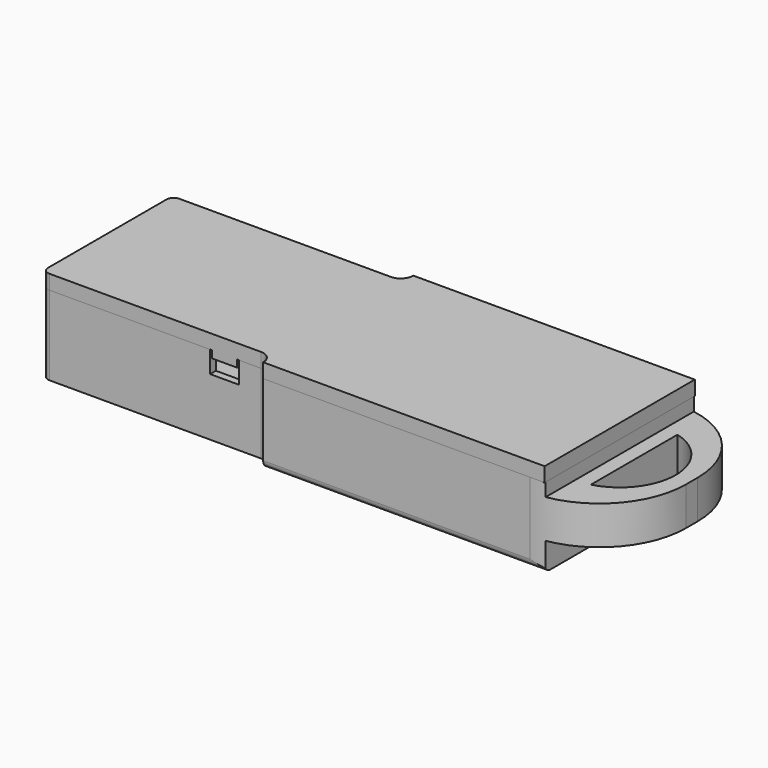
from build123d import *

# Parameters (mm, degrees)
F0_W         = 31
F0_H         = 17.5
F0_W_2       = 1
F1_DEPTH     = 8.5
F2_T         = 2.5
F3_W         = 1
F3_H         = 1
F4_DEPTH     = 6.5
F5_R         = 1
F6_W         = 9.5
F6_H         = 6
F8_DEPTH     = 1.5
F7_W         = 4
F7_H         = 4
F9_DEPTH     = 2
F11_DEPTH    = 2
F13_DEPTH    = 2
F14_R        = 1
F15_R        = 1.7
F15_2_R      = 1.7
F17_DEPTH    = 1.75
F18_W        = 12.5
F18_H        = 7.25
F19_DEPTH    = 3
F20_W        = 1.25
F20_H        = 12
F21_DEPTH    = 2.25
F22_W        = 3.5
F22_H        = 1
F23_DEPTH    = 1
F24_W        = 1
F24_H        = 4
F25_DEPTH    = 2
F26_W        = 2
F26_H        = 4
F27_DEPTH    = 1
F28_SIZE     = 0.99999
F29_W        = 6
F29_H        = 2
F30_DEPTH    = 0.25
F32_DEPTH    = 10
F33_T1_DEPTH = 65.3331902927
F35_DEPTH    = 10


# Not quite as in the source:
# - a fillet or chamfer that OpenCascade refuses, or shapes differently, is made with other operations: its cross-section is extruded or revolved along the edge and cut away or added
# - a fillet or chamfer is up to 0.001 mm smaller than in the source, because OpenCascade refuses the exact size


with BuildPart() as f1:
    # F0 (on Top) → F1 (new body)
    with BuildSketch(Plane.XY):
        Rectangle(F0_W, F0_H)
        with Locations((16, 0)):
            Rectangle(F0_W_2, F0_H)
        Polygon((16.5, 10.5), (16.5, 8.75), (16.5, -8.75), (16.5, -10.5), (50.5, -10.5), (50.5, 10.5), align=None)
    extrude(amount=F1_DEPTH)

    # F2
    f2_openings = [f1.faces().sort_by_distance(p)[0] for p in [
        (18.994505, 0, 8.5),
    ]]
    offset(amount=F2_T, openings=f2_openings, kind=Kind.INTERSECTION)

    # F3 (on face) → F4 (join)
    with BuildSketch(Plane.XY):
        with Locations((16, 4.5)):
            Rectangle(F3_W, F3_H)
        with Locations((16, 1.5)):
            Rectangle(F3_W, F3_H)
        with Locations((16, -1.5)):
            Rectangle(F3_W, F3_H)
        with Locations((16, -4.5)):
            Rectangle(F3_W, F3_H)
    extrude(amount=F4_DEPTH)

    # F5
    f5_edges = [f1.edges().sort_by_distance(p)[0] for p in [
        (-18, 11.25, 3),
        (-18, -11.25, 3),
        (33.5, -13, -2.5),
        (33.5, 13, -2.5),
    ]]
    fillet(f5_edges, radius=F5_R)

    # F6 (on face) → F8 (cut, symmetric)
    with BuildSketch(Plane(origin=(0, -8.75, 0), x_dir=(-1, 0, 0), z_dir=(0, 1, 0))):
        with Locations((-7.25, 7.5)):
            Rectangle(F6_W, F6_H)
    extrude(amount=F8_DEPTH, both=True, mode=Mode.SUBTRACT)

    # F7 (on face) → F9 (cut, symmetric)
    with BuildSketch(Plane.XZ.offset(11.25)):
        with Locations((7.25, 7.5)):
            Rectangle(F7_W, F7_H)
    extrude(amount=F9_DEPTH, both=True, mode=Mode.SUBTRACT)

    # F10 (on face) → F11 (cut)
    with BuildSketch(Plane.XY.offset(8.5)):
        Polygon((2.5, -8.75), (-15.5, -8.75), (-15.5, 8.75), (15.5, 8.75), (15.5, 10), (-16.75, 10), (-16.75, 8.75), (-16.75, -10), (2.5, -10), align=None)
        Polygon((15.5, 10), (15.5, 8.75), (16.5, 8.75), (16.5, 10.5), (50.5, 10.5), (50.5, -10.5), (16.5, -10.5), (16.5, -8.75), (12, -8.75), (12, -10), (15.5, -10), (15.5, -11.75), (16.5, -11.75), (51.75, -11.75), (51.75, 10.5), (51.75, 11.75), (50.5, 11.75), (16.5, 11.75), (15.5, 11.75), align=None)
    extrude(amount=-F11_DEPTH, mode=Mode.SUBTRACT)

    # F15#2
    f15_2_edges = [f1.edges().sort_by_distance(p)[0] for p in [
        (14, 11.25, 3),
        (14, -11.25, 3),
    ]]
    fillet(f15_2_edges, radius=F15_2_R)


with BuildPart() as f13:
    # F12 (on face) → F13 (new body)
    with BuildSketch(Plane.XY.offset(8.5)):
        Polygon((14, 11.25), (-18, 11.25), (-18, -11.25), (14, -11.25), (14, -13), (53, -13), (53, 13), (14, 13), align=None)
    extrude(amount=F13_DEPTH)

    # F14
    f14_edges = [f13.edges().sort_by_distance(p)[0] for p in [
        (-18, 11.25, 9.5),
        (-18, -11.25, 9.5),
    ]]
    fillet(f14_edges, radius=F14_R)

    # F15
    f15_edges = [f13.edges().sort_by_distance(p)[0] for p in [
        (14, -11.25, 9.5),
        (14, 11.25, 9.5),
    ]]
    fillet(f15_edges, radius=F15_R)

    # F16 (on face) → F17 (join)
    with BuildSketch(Plane(origin=(0, 0, 8.5), x_dir=(1, 0, 0), z_dir=(0, 0, -1))):
        Polygon((-15.5, -9.75), (-15.5, -8.75), (-15.5, 8.75), (2.5, 8.75), (2.5, 9.75), (-16.5, 9.75), (-16.5, -9.75), align=None)
        Polygon((16.5, -8.75), (-15.5, -8.75), (-15.5, -9.75), (15.75, -9.75), (15.75, -11.5), (51.5, -11.5), (51.5, 11.5), (16.5, 11.5), (15.75, 11.5), (15.75, 9.75), (12, 9.75), (12, 8.75), (16.5, 8.75), (16.5, 10.5), (50.5, 10.5), (50.5, -10.5), (16.5, -10.5), align=None)
    extrude(amount=F17_DEPTH)


with BuildPart() as f19_tool:
    # F18 (on face) → F19 (new body)
    with BuildSketch(Plane(origin=(-18, 0, 0), x_dir=(0, -1, 0), z_dir=(-1, 0, 0))):
        with Locations((0, 4.875)):
            Rectangle(F18_W, F18_H)
    extrude(amount=-F19_DEPTH)


with BuildPart() as f1_1:
    add(f1.part)

    # F19: cut by f19_tool
    add(f19_tool.part, mode=Mode.SUBTRACT)

    # F31 (on face) → F32 (join)
    with BuildSketch(Plane.YZ.offset(53)):
        Polygon((-13, 1.3334048537), (13, 1.3334048537), (13, 6.6665951463), (0, 6.6665951463), (-13, 6.6665951463), align=None)
    extrude(amount=F32_DEPTH)

    # F33: fillet of radius 12 on 2 edges, made by hand

    # F33_s2 → F33_t1 (cut)
    with BuildSketch(Plane.XY.offset(-28.6665951463)):
        with BuildLine():
            ThreePointArc((51, -13), (59.4852813742, -9.4852813742), (63, -1))
            Line((63, -1), (63, -13))
            Line((63, -13), (51, -13))
        make_face()
        with BuildLine():
            ThreePointArc((51, 13), (59.4852813742, 9.4852813742), (63, 1))
            Line((63, 1), (63, 13))
            Line((63, 13), (51, 13))
        make_face()
    extrude(amount=F33_T1_DEPTH, mode=Mode.SUBTRACT)

    # F34 (on face) → F35 (cut, symmetric)
    with BuildSketch(Plane.XY.offset(6.6665951463)):
        with BuildLine():
            Line((55, 0), (55, -7.5))
            ThreePointArc((55, -7.5), (60.7620873481, 0), (55, 7.5))
            Line((55, 7.5), (55, 0))
        make_face()
    extrude(amount=F35_DEPTH, both=True, mode=Mode.SUBTRACT)


with BuildPart() as f13_1:
    add(f13.part)

    # F19: cut by f19_tool
    add(f19_tool.part, mode=Mode.SUBTRACT)

    # F20 (on face) → F21 (join)
    with BuildSketch(Plane.XY.offset(8.5)):
        with Locations((-17.375, 0)):
            Rectangle(F20_W, F20_H)
    extrude(amount=-F21_DEPTH)

    # F22 (on face) → F23 (join)
    with BuildSketch(Plane(origin=(0, 0, 8.5), x_dir=(1, 0, 0), z_dir=(0, 0, -1))):
        with Locations((7.25, 10.75)):
            Rectangle(F22_W, F22_H)
    extrude(amount=F23_DEPTH)

    # F24 (on face) → F25 (join)
    with BuildSketch(Plane(origin=(0, -8.75, 0), x_dir=(-1, 0, 0), z_dir=(0, 1, 0))):
        with Locations((-2, 6.5)):
            Rectangle(F24_W, F24_H)
        with Locations((-12.5, 6.5)):
            Rectangle(F24_W, F24_H)
    extrude(amount=F25_DEPTH)

    # F26 (on face) → F27 (join)
    with BuildSketch(Plane(origin=(0, -6.75, 0), x_dir=(-1, 0, 0), z_dir=(0, 1, 0))):
        with Locations((-2.5, 6.5)):
            Rectangle(F26_W, F26_H)
        with Locations((-12, 6.5)):
            Rectangle(F26_W, F26_H)
    extrude(amount=F27_DEPTH)

    # F28 (size 1 in the source; OpenCascade refuses exactly that, so slightly less here)
    f28_edges = [f13_1.edges().sort_by_distance(p)[0] for p in [
        (3.5, -5.75, 6.5),
        (11, -5.75, 6.5),
    ]]
    chamfer(f28_edges, length=F28_SIZE)

    # F29 (on face) → F30 (join)
    with BuildSketch(Plane(origin=(0, 0, 8.5), x_dir=(1, 0, 0), z_dir=(0, 0, -1))):
        with Locations((-13.75, -5)):
            Rectangle(F29_W, F29_H)
        with Locations((-13.75, 5)):
            Rectangle(F29_W, F29_H)
    extrude(amount=F30_DEPTH)


solid = Compound([f1_1.part, f13_1.part])
